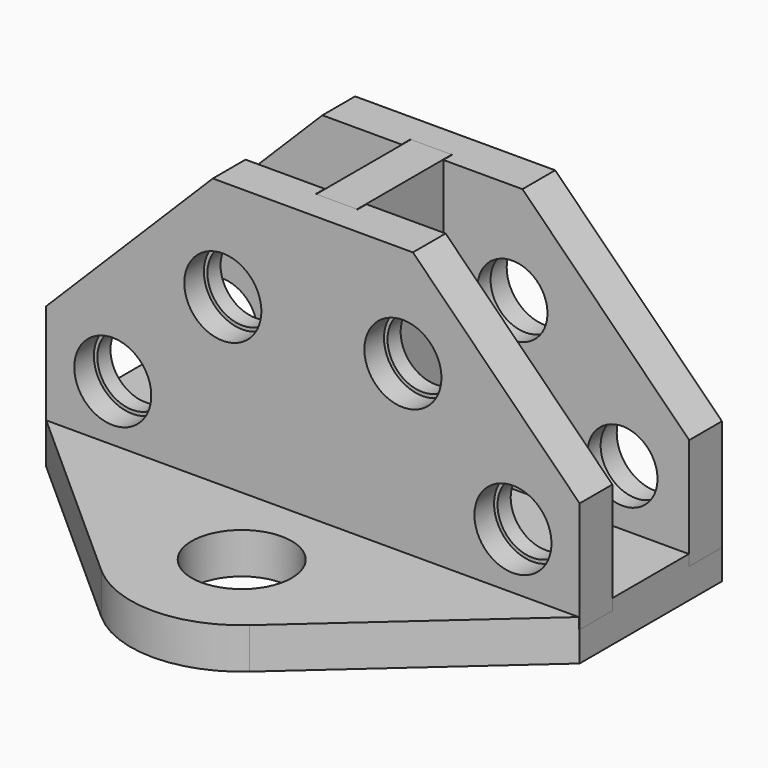
from build123d import *

# Parameters (mm, degrees)
F0_R      = 14.2875
F1_DEPTH  = 11.684
F3_DEPTH  = 11.684
F4_R      = 11
F5_DEPTH  = 7
F6_R      = 10
F7_DEPTH  = 4.684
F13_W     = 11.684
F13_H     = 33.782
F14_DEPTH = 79.375
F16_DEPTH = 3.175
F17_W     = 11.938
F17_H     = 33.782
F18_DEPTH = 79.375


with BuildPart() as f1:
    # F0 (on Top) → F1 (new body)
    with BuildSketch(Plane.XY):
        with BuildLine():
            Line((-76.2, 25.4), (-21.1287915932, -23.6988747795))
            ThreePointArc((-21.1287915932, -23.6988747795), (0, -31.75), (21.1287915932, -23.6988747795))
            Line((21.1287915932, -23.6988747795), (76.2, 25.4))
            Line((76.2, 25.4), (76.2, 76.2))
            Line((76.2, 76.2), (-76.2, 76.2))
            Line((-76.2, 76.2), (-76.2, 25.4))
        make_face()
        Circle(F0_R, mode=Mode.SUBTRACT)
    extrude(amount=F1_DEPTH)

    # F15 (on face) → F16 (cut, through all)
    with BuildSketch(Plane.XY.offset(11.684)):
        Polygon((76.2, 76.2), (-76.2, 76.2), (-76.2, 64.389), (-5.969, 64.389), (-5.969, 37.211), (-76.2, 37.211), (-76.2, 25.273), (76.2, 25.273), (76.2, 37.211), (5.969, 37.211), (5.969, 64.389), (76.2, 64.389), align=None)
    extrude(amount=-F16_DEPTH, mode=Mode.SUBTRACT)


with BuildPart() as f3:
    # F2 (on face) → F3 (new body)
    with BuildSketch(Plane(origin=(0, 76.2, 0), x_dir=(-1, 0, 0), z_dir=(0, 1, 0))):
        Polygon((-76.2, 40.259), (-76.2, 8.509), (76.2, 8.509), (76.2, 40.259), (28.575, 87.884), (-28.575, 87.884), align=None)
    extrude(amount=-F3_DEPTH)

    # F4 (on face) → F5 (cut)
    with BuildSketch(Plane(origin=(0, 76.2, 0), x_dir=(-1, 0, 0), z_dir=(0, 1, 0))):
        with Locations((-57.15, 27.559)):
            Circle(F4_R)
        with Locations((-25.7191035763, 58.9898964237)):
            Circle(F4_R)
        with Locations((25.7191035763, 58.9898964237)):
            Circle(F4_R)
        with Locations((57.15, 27.559)):
            Circle(F4_R)
    extrude(amount=-F5_DEPTH, mode=Mode.SUBTRACT)

    # F6 (on face) → F7 (cut, through all)
    with BuildSketch(Plane(origin=(0, 69.2, 0), x_dir=(-1, 0, 0), z_dir=(0, 1, 0))):
        with Locations((-25.7191035763, 58.9898964237)):
            Circle(F6_R)
        with Locations((-57.15, 27.559)):
            Circle(F6_R)
        with Locations((25.7191035763, 58.9898964237)):
            Circle(F6_R)
        with Locations((57.15, 27.559)):
            Circle(F6_R)
    extrude(amount=-F7_DEPTH, mode=Mode.SUBTRACT)


with BuildPart() as f12_1:
    # F12: instance of F3
    add(f3.part.mirror(Plane(origin=(-76.2, 50.8, 11.684), x_dir=(0, 0, -1), z_dir=(0, 1, 0))))


with BuildPart() as f14:
    # F13 (on face) → F14 (new body, through all)
    with BuildSketch(Plane.XY.offset(87.884)):
        with Locations((0, 50.8)):
            Rectangle(F13_W, F13_H)
    extrude(amount=-F14_DEPTH)


with BuildPart() as f18_tool:
    # F17 (on face) → F18 (new body, through all)
    with BuildSketch(Plane.XY.offset(87.884)):
        with Locations((0, 50.8)):
            Rectangle(F17_W, F17_H)
    extrude(amount=-F18_DEPTH)


with BuildPart() as f3_1:
    add(f3.part)

    # F18: cut by f18_tool
    add(f18_tool.part, mode=Mode.SUBTRACT)


with BuildPart() as f12_1_1:
    add(f12_1.part)

    # F18: cut by f18_tool
    add(f18_tool.part, mode=Mode.SUBTRACT)


solid = Compound([f1.part, f14.part, f3_1.part, f12_1_1.part])
